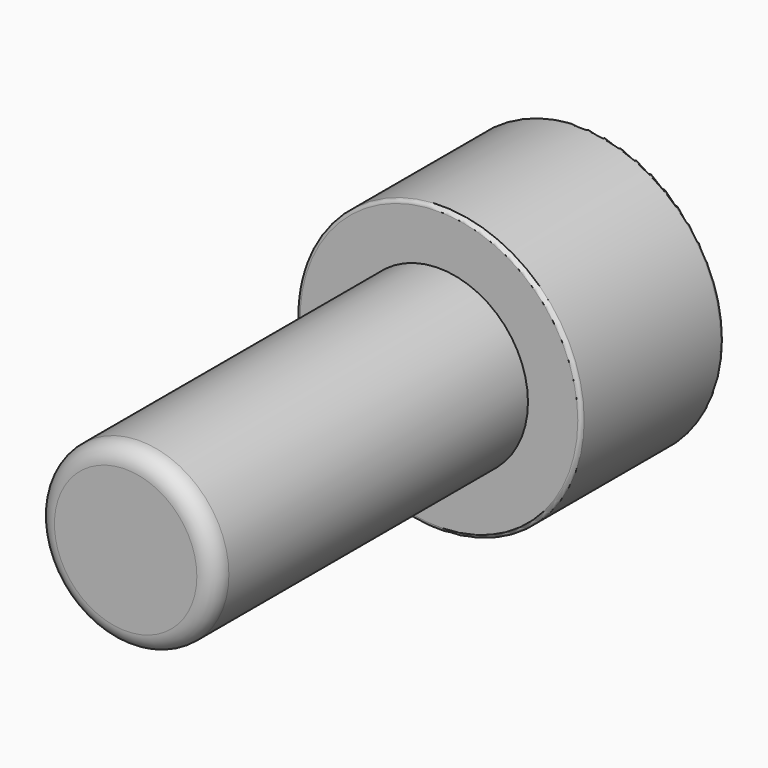
from build123d import *

# Parameters (mm, degrees)
F0_R     = 5
F1_DEPTH = 22
F0_R_2   = 8
F2_DEPTH = 10
F4_DEPTH = 8
F5_R     = 0.2
F6_R     = 1


# Not quite as in the source:
# - a feature names something its author has since deleted; it is built from what else it names


with BuildPart() as f1:
    # F0 (on Front) → F1 (new body)
    with BuildSketch(Plane.XZ):
        Circle(F0_R)
    extrude(amount=F1_DEPTH)

    # F0 (on Front) → F2 (join)
    with BuildSketch(Plane.XZ):
        Circle(F0_R_2)
        Circle(F0_R, mode=Mode.SUBTRACT)
        Circle(F0_R)
    extrude(amount=-F2_DEPTH)

    # F3 (on face) → F4 (cut)
    with BuildSketch(Plane(origin=(0, 10, 0), x_dir=(-1, 0, 0), z_dir=(0, 1, 0))):
        Polygon((-2.3094010768, -4), (2.3094010768, -4), (4.6188021535, 0), (2.3094010768, 4), (-2.3094010768, 4), (-4.6188021535, 0), align=None)
    extrude(amount=-F4_DEPTH, mode=Mode.SUBTRACT)

    # F5
    f5_edges = [f1.edges().sort_by_distance(p)[0] for p in [
        (-3.464102, 2, 2),
        (3.464102, 2, -2),
        (0, 2, 4),
        (0, 10, -4),
        (-3.464102, 2, -2),
        (0, 2, -4),
        (3.464102, 10, 2),
        (3.464102, 2, 2),
        (-3.464102, 10, -2),
        (-3.464102, 10, 2),
        (-8, 10, 0),
        (0, 10, 4),
        (3.464102, 10, -2),
        (-8, 0, 0),
    ]]
    fillet(f5_edges, radius=F5_R)

    # F6
    f6_edges = [f1.edges().sort_by_distance(p)[0] for p in [
        (-5, -22, 0),
    ]]
    fillet(f6_edges, radius=F6_R)


solid = f1.part
